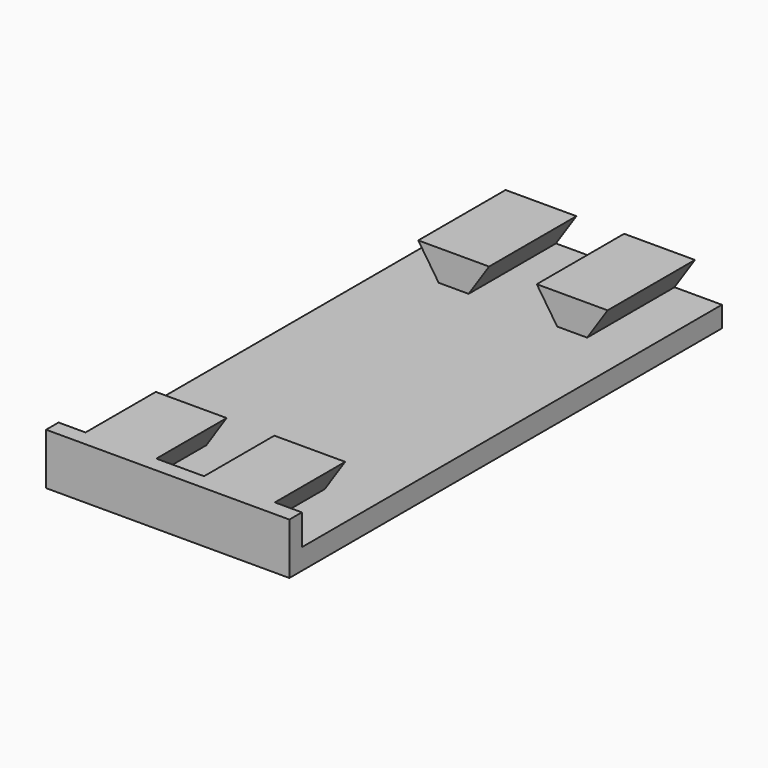
from build123d import *

# Parameters (mm, degrees)
F0_W     = 23.4
F0_H     = 52
F1_DEPTH = 2
F3_START = 15.05
F3_DEPTH = 9.95
F4_W     = 4.5600925213
F4_H     = 1.5
F4_W_2   = 8.5201850425
F5_DEPTH = 2.95
F6_START = -16.5
F6_DEPTH = 10.5


with BuildPart() as f1:
    # F0 (on Top) → F1 (new body)
    with BuildSketch(Plane.XY):
        with Locations((0, 1)):
            Rectangle(F0_W, F0_H)
    extrude(amount=F1_DEPTH)

    # F2 (on Front) → F3 (join)
    with BuildSketch(Plane.XZ.offset(F3_START)):
        Polygon((2.2934258546, 4.95), (4.2600925213, 2), (7.1399074787, 2), (9.1065741454, 4.95), align=None)
        Polygon((-4.2600925213, 2), (-2.2934258546, 4.95), (-9.1065741454, 4.95), (-7.1399074787, 2), align=None)
    extrude(amount=F3_DEPTH)

    # F4 (on face) → F5 (join)
    with BuildSketch(Plane.XY.offset(2)):
        with Locations((9.4199537394, -24.25)):
            Rectangle(F4_W, F4_H)
        with Locations((0, -24.25)):
            Rectangle(F4_W_2, F4_H)
        with Locations((-9.4199537394, -24.25)):
            Rectangle(F4_W, F4_H)
    extrude(amount=F5_DEPTH)

    # F2 (on Front) → F6 (join)
    with BuildSketch(Plane.XZ.offset(F6_START)):
        Polygon((2.2934258546, 4.95), (4.2600925213, 2), (7.1399074787, 2), (9.1065741454, 4.95), align=None)
        Polygon((-4.2600925213, 2), (-2.2934258546, 4.95), (-9.1065741454, 4.95), (-7.1399074787, 2), align=None)
    extrude(amount=-F6_DEPTH)


solid = f1.part
